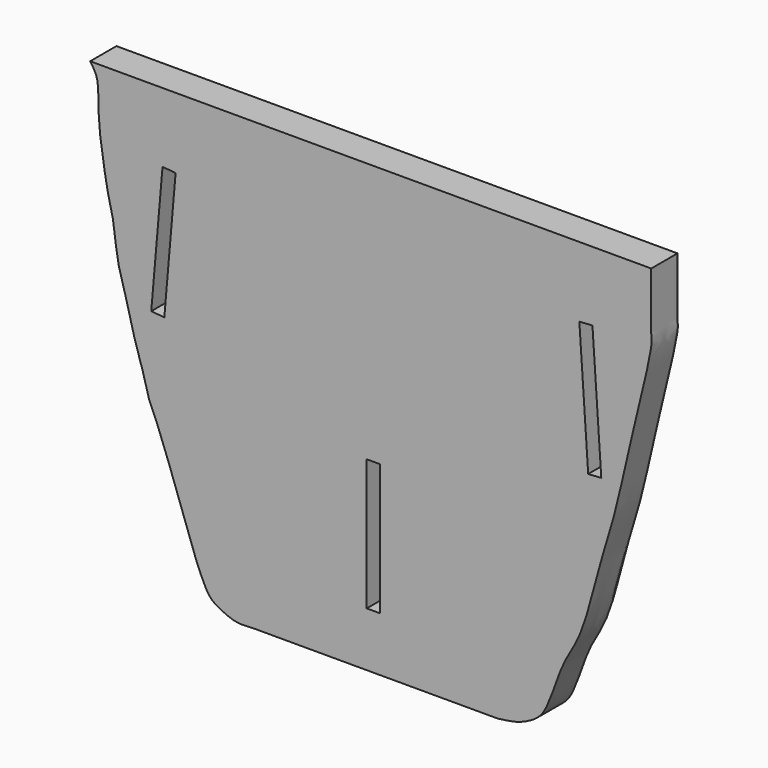
from build123d import *

# Parameters (mm, degrees)
F1_DEPTH = 1
F2_DEPTH = 30


# Not quite as in the source:
# - a feature names something its author has since deleted; it is built from what else it names


with BuildPart() as f1:
    # F0 (on Front) → F1 (new body)
    with BuildSketch(Plane.XZ):
        with BuildLine():
            add(Edge.make_bspline(
                [(425.694167614, 314.9593174458), (425.7411635664, 306.5823239179), (425.8353031998, 289.8020043845), (425.2213058119, 260.8518364023), (427.5387063586, 252.1953752472), (403.8651896897, 159.3760040825), (394.9399909924, 115.0243838579), (383.5203150006, 76.7031238113), (377.471464527, 57.9641754851), (362.9083470803, -2.5900933423), (345.2420278931, -25.5103393777), (334.7762850188, -58.8866961253), (326.7161367987, -76.5853711865), (317.2191947156, -83.9165976747), (303.6744184479, -90.5988549349), (291.5596455088, -92.0742269797), (285.1151227951, -92.8590595722)],
                knots=[0, 0, 0, 0, 0.0678721046, 0.1359575603, 0.1770145832, 0.3026200399, 0.39906864, 0.477401143, 0.5385059508, 0.6402294069, 0.7140746489, 0.7906886976, 0.8481181215, 0.8921936726, 0.9426518079, 1, 1, 1, 1], degree=3))
            Line((425.694167614, 314.9593174458), (-87.1654751293, 314.9593174458))
            add(Edge.make_bspline(
                [(62.4156631529, -92.8590595722), (57.0412799038, -93.2430841848), (46.7781604835, -93.9764316735), (34.762824297, -88.8868818229), (23.1000241889, -83.0505840006), (16.6656980071, -71.5759104343), (9.2152702261, -54.4172118892), (3.6540691421, -37.3377357492), (-3.596042902, -17.563668233), (-9.9992245943, -0.2210912492), (-16.1877714037, 17.9491344863), (-22.3081726097, 32.6077543724), (-26.6364419857, 45.9390385377), (-33.8295661577, 58.8731002038), (-38.5610064547, 81.4119978236), (-45.5627001907, 99.3824651482), (-50.8940688236, 123.5390915977), (-56.5692018159, 142.1363827936), (-60.9443389374, 157.495862805), (-63.7160996981, 172.3778561971), (-65.4868817968, 193.5985919764), (-70.5111342627, 211.0693794771), (-73.6652423642, 228.9065774682), (-78.0528125256, 255.4192638339), (-80.2249024033, 280.7772367064), (-79.1591451026, 303.4353757219), (-84.7282168765, 311.4512404644), (-87.1654751293, 314.9593174458)],
                knots=[0, 0, 0, 0, 0.0371469817, 0.070937239, 0.1041076852, 0.1377363763, 0.1783245219, 0.2187259528, 0.2617260214, 0.3025703504, 0.3437531553, 0.3813536818, 0.4160576409, 0.4522458314, 0.496957828, 0.5390308214, 0.5856683097, 0.6275330442, 0.6645798021, 0.7012650834, 0.7446384462, 0.7847130572, 0.8246319824, 0.8733648148, 0.9218849639, 0.9658135998, 1, 1, 1, 1], degree=3))
            Line((62.4156631529, -92.8590595722), (285.1151227951, -92.8590595722))
        make_face()
        Polygon((165.6303541942, 76.8693466235), (171.6303541942, 76.8693466235), (177.6303541942, 76.8693466235), (177.6303541942, -43.1306533765), (171.6303541942, -43.1306533765), (165.6303541942, -43.1306533765), align=None, mode=Mode.SUBTRACT)
        Polygon((-31.3533060253, 131.947606802), (-21.0363371185, 251.5032848461), (-9.0807693141, 250.4715879554), (-19.3977382209, 130.9159099113), align=None, mode=Mode.SUBTRACT)
        Polygon((359.9782669565, 250.8293367838), (371.9512232727, 251.634518161), (380.0212239228, 131.634518161), (368.0482676066, 130.8293367838), align=None, mode=Mode.SUBTRACT)
    extrude(amount=F1_DEPTH)

    # F0 (on Front) → F2 (join)
    with BuildSketch(Plane.XZ):
        with BuildLine():
            add(Edge.make_bspline(
                [(425.694167614, 314.9593174458), (425.7411635664, 306.5823239179), (425.8353031998, 289.8020043845), (425.2213058119, 260.8518364023), (427.5387063586, 252.1953752472), (403.8651896897, 159.3760040825), (394.9399909924, 115.0243838579), (383.5203150006, 76.7031238113), (377.471464527, 57.9641754851), (362.9083470803, -2.5900933423), (345.2420278931, -25.5103393777), (334.7762850188, -58.8866961253), (326.7161367987, -76.5853711865), (317.2191947156, -83.9165976747), (303.6744184479, -90.5988549349), (291.5596455088, -92.0742269797), (285.1151227951, -92.8590595722)],
                knots=[0, 0, 0, 0, 0.0678721046, 0.1359575603, 0.1770145832, 0.3026200399, 0.39906864, 0.477401143, 0.5385059508, 0.6402294069, 0.7140746489, 0.7906886976, 0.8481181215, 0.8921936726, 0.9426518079, 1, 1, 1, 1], degree=3))
            Line((425.694167614, 314.9593174458), (-87.1654751293, 314.9593174458))
            add(Edge.make_bspline(
                [(62.4156631529, -92.8590595722), (57.0412799038, -93.2430841848), (46.7781604835, -93.9764316735), (34.762824297, -88.8868818229), (23.1000241889, -83.0505840006), (16.6656980071, -71.5759104343), (9.2152702261, -54.4172118892), (3.6540691421, -37.3377357492), (-3.596042902, -17.563668233), (-9.9992245943, -0.2210912492), (-16.1877714037, 17.9491344863), (-22.3081726097, 32.6077543724), (-26.6364419857, 45.9390385377), (-33.8295661577, 58.8731002038), (-38.5610064547, 81.4119978236), (-45.5627001907, 99.3824651482), (-50.8940688236, 123.5390915977), (-56.5692018159, 142.1363827936), (-60.9443389374, 157.495862805), (-63.7160996981, 172.3778561971), (-65.4868817968, 193.5985919764), (-70.5111342627, 211.0693794771), (-73.6652423642, 228.9065774682), (-78.0528125256, 255.4192638339), (-80.2249024033, 280.7772367064), (-79.1591451026, 303.4353757219), (-84.7282168765, 311.4512404644), (-87.1654751293, 314.9593174458)],
                knots=[0, 0, 0, 0, 0.0371469817, 0.070937239, 0.1041076852, 0.1377363763, 0.1783245219, 0.2187259528, 0.2617260214, 0.3025703504, 0.3437531553, 0.3813536818, 0.4160576409, 0.4522458314, 0.496957828, 0.5390308214, 0.5856683097, 0.6275330442, 0.6645798021, 0.7012650834, 0.7446384462, 0.7847130572, 0.8246319824, 0.8733648148, 0.9218849639, 0.9658135998, 1, 1, 1, 1], degree=3))
            Line((62.4156631529, -92.8590595722), (285.1151227951, -92.8590595722))
        make_face()
        Polygon((165.6303541942, 76.8693466235), (171.6303541942, 76.8693466235), (177.6303541942, 76.8693466235), (177.6303541942, -43.1306533765), (171.6303541942, -43.1306533765), (165.6303541942, -43.1306533765), align=None, mode=Mode.SUBTRACT)
        Polygon((-31.3533060253, 131.947606802), (-21.0363371185, 251.5032848461), (-9.0807693141, 250.4715879554), (-19.3977382209, 130.9159099113), align=None, mode=Mode.SUBTRACT)
        Polygon((359.9782669565, 250.8293367838), (371.9512232727, 251.634518161), (380.0212239228, 131.634518161), (368.0482676066, 130.8293367838), align=None, mode=Mode.SUBTRACT)
    extrude(amount=F2_DEPTH)


solid = f1.part
